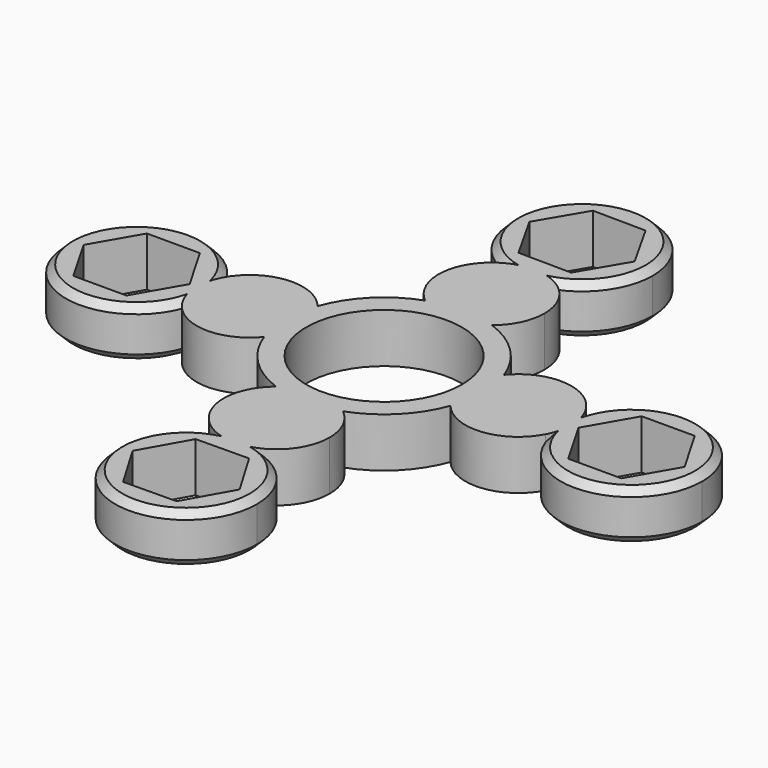
from build123d import *

# Parameters (mm, degrees)
F0_R         = 11
F1_DEPTH     = 7
F2_T4_ANGLE  = 348.6337760753
F2_S5_R      = 7.5
F2_T6_DEPTH  = 16
F2_T10_ANGLE = 348.6337760753
F2_S11_R     = 7.5
F2_T12_DEPTH = 16
F2_T16_ANGLE = 348.6337760753
F2_S17_R     = 7.5
F2_T18_DEPTH = 16
F2_T22_ANGLE = 348.6337760753
F2_S23_R     = 7.5
F2_T24_DEPTH = 16
F3_T4_ANGLE  = 348.6337760753
F3_S5_R      = 7.5
F3_T6_DEPTH  = 16
F3_T10_ANGLE = 348.6337760753
F3_S11_R     = 7.5
F3_T12_DEPTH = 16
F3_T16_ANGLE = 348.6337760753
F3_S17_R     = 7.5
F3_T18_DEPTH = 16
F3_T22_ANGLE = 348.6337760753
F3_S23_R     = 7.5
F3_T24_DEPTH = 16


# Not quite as in the source:
# - a fillet or chamfer that OpenCascade refuses, or shapes differently, is made with other operations: its cross-section is extruded or revolved along the edge and cut away or added


with BuildPart() as f1:
    # F0 (on Top) → F1 (new body)
    with BuildSketch(Plane.XY):
        with BuildLine():
            ThreePointArc((13.1776315789, -4.727581408), (13.7928757354, -2.3992871748), (14, 0))
            ThreePointArc((14, 0), (13.7928757354, 2.3992871748), (13.1776315789, 4.727581408))
            ThreePointArc((13.1776315789, 4.727581408), (11.5, 0), (13.1776315789, -4.727581408))
        make_face()
        with BuildLine():
            ThreePointArc((13.1776315789, 4.727581408), (13.7928757354, 2.3992871748), (14, 0))
            ThreePointArc((14, 0), (13.7928757354, -2.3992871748), (13.1776315789, -4.727581408))
            ThreePointArc((13.1776315789, -4.727581408), (19.7351433448, -7.4638839931), (25.6328125, -3.5008282363))
            ThreePointArc((25.6328125, -3.5008282363), (25, 0), (25.6328125, 3.5008282363))
            ThreePointArc((25.6328125, 3.5008282363), (19.7351433448, 7.4638839931), (13.1776315789, 4.727581408))
        make_face()
        with BuildLine():
            ThreePointArc((13.1776315789, -4.727581408), (11.5, 0), (13.1776315789, 4.727581408))
            ThreePointArc((13.1776315789, 4.727581408), (9.8994949366, 9.8994949366), (4.727581408, 13.1776315789))
            ThreePointArc((4.727581408, 13.1776315789), (0, 11.5), (-4.727581408, 13.1776315789))
            ThreePointArc((-4.727581408, 13.1776315789), (-9.8994949366, 9.8994949366), (-13.1776315789, 4.727581408))
            ThreePointArc((-13.1776315789, 4.727581408), (-11.9318402976, 2.5082102027), (-11.5, 0))
            ThreePointArc((-11.5, 0), (-11.9318402976, -2.5082102027), (-13.1776315789, -4.727581408))
            ThreePointArc((-13.1776315789, -4.727581408), (-9.8994949366, -9.8994949366), (-4.727581408, -13.1776315789))
            ThreePointArc((-4.727581408, -13.1776315789), (0, -11.5), (4.727581408, -13.1776315789))
            ThreePointArc((4.727581408, -13.1776315789), (9.8994949366, -9.8994949366), (13.1776315789, -4.727581408))
        make_face()
        Circle(F0_R, mode=Mode.SUBTRACT)
        with BuildLine():
            ThreePointArc((-4.727581408, 13.1776315789), (0, 11.5), (4.727581408, 13.1776315789))
            ThreePointArc((4.727581408, 13.1776315789), (0, 14), (-4.727581408, 13.1776315789))
        make_face()
        with BuildLine():
            ThreePointArc((-4.727581408, 13.1776315789), (0, 14), (4.727581408, 13.1776315789))
            ThreePointArc((4.727581408, 13.1776315789), (6.7715160991, 15.7756287869), (7.5, 19))
            ThreePointArc((7.5, 19), (6.4228580777, 22.8725823573), (3.5008282363, 25.6328125))
            ThreePointArc((3.5008282363, 25.6328125), (0, 25), (-3.5008282363, 25.6328125))
            ThreePointArc((-3.5008282363, 25.6328125), (-7.4638839931, 19.7351433448), (-4.727581408, 13.1776315789))
        make_face()
        with BuildLine():
            ThreePointArc((45, 0), (36.7787811838, 9.8405252655), (25.6328125, 3.5008282363))
            ThreePointArc((25.6328125, 3.5008282363), (26.2799757469, 1.8033172558), (26.5, 0))
            ThreePointArc((26.5, 0), (26.2799757469, -1.8033172558), (25.6328125, -3.5008282363))
            ThreePointArc((25.6328125, -3.5008282363), (36.7787811838, -9.8405252655), (45, 0))
        make_face()
        Polygon((31.2446139721, 6.4984928341), (38.7501668667, 6.5015061182), (42.5055528946, 0.0030132841), (38.7553860279, -6.4984928341), (31.2498331333, -6.5015061182), (27.4944471054, -0.0030132841), align=None, mode=Mode.SUBTRACT)
        with BuildLine():
            ThreePointArc((26.5, 0), (26.2799757469, 1.8033172558), (25.6328125, 3.5008282363))
            ThreePointArc((25.6328125, 3.5008282363), (25, 0), (25.6328125, -3.5008282363))
            ThreePointArc((25.6328125, -3.5008282363), (26.2799757469, -1.8033172558), (26.5, 0))
        make_face()
        with BuildLine():
            ThreePointArc((7.5, -19), (6.7715160991, -15.7756287869), (4.727581408, -13.1776315789))
            ThreePointArc((4.727581408, -13.1776315789), (0, -14), (-4.727581408, -13.1776315789))
            ThreePointArc((-4.727581408, -13.1776315789), (-7.4638839931, -19.7351433448), (-3.5008282363, -25.6328125))
            ThreePointArc((-3.5008282363, -25.6328125), (0, -25), (3.5008282363, -25.6328125))
            ThreePointArc((3.5008282363, -25.6328125), (6.4228580777, -22.8725823573), (7.5, -19))
        make_face()
        with BuildLine():
            ThreePointArc((-4.727581408, -13.1776315789), (0, -14), (4.727581408, -13.1776315789))
            ThreePointArc((4.727581408, -13.1776315789), (0, -11.5), (-4.727581408, -13.1776315789))
        make_face()
        with BuildLine():
            ThreePointArc((-11.5, 0), (-11.9318402976, 2.5082102027), (-13.1776315789, 4.727581408))
            ThreePointArc((-13.1776315789, 4.727581408), (-14, 0), (-13.1776315789, -4.727581408))
            ThreePointArc((-13.1776315789, -4.727581408), (-11.9318402976, -2.5082102027), (-11.5, 0))
        make_face()
        with BuildLine():
            ThreePointArc((-13.1776315789, -4.727581408), (-14, 0), (-13.1776315789, 4.727581408))
            ThreePointArc((-13.1776315789, 4.727581408), (-19.7351433448, 7.4638839931), (-25.6328125, 3.5008282363))
            ThreePointArc((-25.6328125, 3.5008282363), (-25.1594747345, 1.7787811838), (-25, 0))
            ThreePointArc((-25, 0), (-25.1594747345, -1.7787811838), (-25.6328125, -3.5008282363))
            ThreePointArc((-25.6328125, -3.5008282363), (-19.7351433448, -7.4638839931), (-13.1776315789, -4.727581408))
        make_face()
        with BuildLine():
            ThreePointArc((10, 35), (-5.7005139083, 43.216090383), (-3.5008282363, 25.6328125))
            ThreePointArc((-3.5008282363, 25.6328125), (0, 26.5), (3.5008282363, 25.6328125))
            ThreePointArc((3.5008282363, 25.6328125), (8.216090383, 29.2994860917), (10, 35))
        make_face()
        Polygon((-3.684923821, 41.5387055115), (3.8202231703, 41.4605903958), (7.5051469914, 34.9218848843), (3.684923821, 28.4612944885), (-3.8202231703, 28.5394096042), (-7.5051469914, 35.0781151157), align=None, mode=Mode.SUBTRACT)
        with BuildLine():
            ThreePointArc((3.5008282363, 25.6328125), (0, 26.5), (-3.5008282363, 25.6328125))
            ThreePointArc((-3.5008282363, 25.6328125), (0, 25), (3.5008282363, 25.6328125))
        make_face()
        with BuildLine():
            ThreePointArc((3.5008282363, -25.6328125), (0, -25), (-3.5008282363, -25.6328125))
            ThreePointArc((-3.5008282363, -25.6328125), (0, -26.5), (3.5008282363, -25.6328125))
        make_face()
        with BuildLine():
            ThreePointArc((3.5008282363, -25.6328125), (0, -26.5), (-3.5008282363, -25.6328125))
            ThreePointArc((-3.5008282363, -25.6328125), (-5.7005139083, -43.216090383), (10, -35))
            ThreePointArc((10, -35), (8.216090383, -29.2994860917), (3.5008282363, -25.6328125))
        make_face()
        Polygon((3.8202231703, -41.4605903958), (-3.684923821, -41.5387055115), (-7.5051469914, -35.0781151157), (-3.8202231703, -28.5394096042), (3.684923821, -28.4612944885), (7.5051469914, -34.9218848843), align=None, mode=Mode.SUBTRACT)
        with BuildLine():
            ThreePointArc((-25, 0), (-25.1594747345, 1.7787811838), (-25.6328125, 3.5008282363))
            ThreePointArc((-25.6328125, 3.5008282363), (-26.5, 0), (-25.6328125, -3.5008282363))
            ThreePointArc((-25.6328125, -3.5008282363), (-25.1594747345, -1.7787811838), (-25, 0))
        make_face()
        with BuildLine():
            ThreePointArc((-25.6328125, -3.5008282363), (-26.5, 0), (-25.6328125, 3.5008282363))
            ThreePointArc((-25.6328125, 3.5008282363), (-45, 0), (-25.6328125, -3.5008282363))
        make_face()
        Polygon((-38.7501668667, 6.5015061182), (-31.2446139721, 6.4984928341), (-27.4944471054, -0.0030132841), (-31.2498331333, -6.5015061182), (-38.7553860279, -6.4984928341), (-42.5055528946, 0.0030132841), align=None, mode=Mode.SUBTRACT)
    extrude(amount=F1_DEPTH)

    # F2: chamfer of 1 on 4 edges, made by hand


with BuildPart() as f2_tool2:
    # F2_s3 → F2_t4 (revolve)
    with BuildSketch(Plane(origin=(-0.3432183296, 3.4488900698, 0), x_dir=(0, 0, 1), z_dir=(0.099026451, -0.9950848014, 0))):
        Polygon((6, 24.8279680496), (7, 25.8279680496), (7, 24.8279680496), align=None)
    revolve(axis=Axis((-35, 0, 7), (0, 0, 1)), revolution_arc=F2_T4_ANGLE)

    # F2_s5 → F2_t6 (cut, symmetric)
    with BuildSketch(Plane.XY.offset(6.5)):
        with Locations((-19, 0)):
            Circle(F2_S5_R)
    extrude(amount=F2_T6_DEPTH, both=True, mode=Mode.SUBTRACT)


with BuildPart() as f1_1:
    add(f1.part)

    # F2_t1: cut F2_tool2
    add(f2_tool2.part, mode=Mode.SUBTRACT)


with BuildPart() as f2_tool8:
    # F2_s9 → F2_t10 (revolve)
    with BuildSketch(Plane(origin=(3.4488900698, 0.3432183296, 0), x_dir=(0, 0, 1), z_dir=(-0.9950848014, -0.099026451, 0))):
        Polygon((6, 24.8279680496), (7, 25.8279680496), (7, 24.8279680496), align=None)
    revolve(axis=Axis((0, 35, 7), (0, 0, 1)), revolution_arc=F2_T10_ANGLE)

    # F2_s11 → F2_t12 (cut, symmetric)
    with BuildSketch(Plane.XY.offset(6.5)):
        with Locations((0, 19)):
            Circle(F2_S11_R)
    extrude(amount=F2_T12_DEPTH, both=True, mode=Mode.SUBTRACT)


with BuildPart() as f1_2:
    add(f1_1.part)

    # F2_t7: cut F2_tool8
    add(f2_tool8.part, mode=Mode.SUBTRACT)


with BuildPart() as f2_tool14:
    # F2_s15 → F2_t16 (revolve)
    with BuildSketch(Plane(origin=(-3.4488900698, -0.3432183296, 0), x_dir=(0, 0, 1), z_dir=(0.9950848014, 0.099026451, 0))):
        Polygon((6, 24.8279680496), (7, 25.8279680496), (7, 24.8279680496), align=None)
    revolve(axis=Axis((0, -35, 7), (0, 0, 1)), revolution_arc=F2_T16_ANGLE)

    # F2_s17 → F2_t18 (cut, symmetric)
    with BuildSketch(Plane.XY.offset(6.5)):
        with Locations((0, -19)):
            Circle(F2_S17_R)
    extrude(amount=F2_T18_DEPTH, both=True, mode=Mode.SUBTRACT)


with BuildPart() as f1_3:
    add(f1_2.part)

    # F2_t13: cut F2_tool14
    add(f2_tool14.part, mode=Mode.SUBTRACT)


with BuildPart() as f2_tool20:
    # F2_s21 → F2_t22 (revolve)
    with BuildSketch(Plane(origin=(0.3432183296, -3.4488900698, 0), x_dir=(0, 0, 1), z_dir=(-0.099026451, 0.9950848014, 0))):
        Polygon((6, 24.8279680496), (7, 25.8279680496), (7, 24.8279680496), align=None)
    revolve(axis=Axis((35, 0, 7), (0, 0, 1)), revolution_arc=F2_T22_ANGLE)

    # F2_s23 → F2_t24 (cut, symmetric)
    with BuildSketch(Plane.XY.offset(6.5)):
        with Locations((19, 0)):
            Circle(F2_S23_R)
    extrude(amount=F2_T24_DEPTH, both=True, mode=Mode.SUBTRACT)


with BuildPart() as f1_4:
    add(f1_3.part)

    # F2_t19: cut F2_tool20
    add(f2_tool20.part, mode=Mode.SUBTRACT)

    # F3: chamfer of 1 on 4 edges, made by hand


with BuildPart() as f3_tool2:
    # F3_s3 → F3_t4 (revolve)
    with BuildSketch(Plane(origin=(-0.3432183296, 3.4488900698, 0), x_dir=(0, 0, 1), z_dir=(0.099026451, -0.9950848014, 0))):
        Polygon((0, 25.8279680496), (1, 24.8279680496), (0, 24.8279680496), align=None)
    revolve(axis=Axis((-35, 0, 0), (0, 0, 1)), revolution_arc=F3_T4_ANGLE)

    # F3_s5 → F3_t6 (cut, symmetric)
    with BuildSketch(Plane.XY.offset(0.5)):
        with Locations((-19, 0)):
            Circle(F3_S5_R)
    extrude(amount=F3_T6_DEPTH, both=True, mode=Mode.SUBTRACT)


with BuildPart() as f1_5:
    add(f1_4.part)

    # F3_t1: cut F3_tool2
    add(f3_tool2.part, mode=Mode.SUBTRACT)


with BuildPart() as f3_tool8:
    # F3_s9 → F3_t10 (revolve)
    with BuildSketch(Plane(origin=(-3.4488900698, -0.3432183296, 0), x_dir=(0, 0, 1), z_dir=(0.9950848014, 0.099026451, 0))):
        Polygon((0, 25.8279680496), (1, 24.8279680496), (0, 24.8279680496), align=None)
    revolve(axis=Axis((0, -35, 0), (0, 0, 1)), revolution_arc=F3_T10_ANGLE)

    # F3_s11 → F3_t12 (cut, symmetric)
    with BuildSketch(Plane.XY.offset(0.5)):
        with Locations((0, -19)):
            Circle(F3_S11_R)
    extrude(amount=F3_T12_DEPTH, both=True, mode=Mode.SUBTRACT)


with BuildPart() as f1_6:
    add(f1_5.part)

    # F3_t7: cut F3_tool8
    add(f3_tool8.part, mode=Mode.SUBTRACT)


with BuildPart() as f3_tool14:
    # F3_s15 → F3_t16 (revolve)
    with BuildSketch(Plane(origin=(0.3432183296, -3.4488900698, 0), x_dir=(0, 0, 1), z_dir=(-0.099026451, 0.9950848014, 0))):
        Polygon((1, 24.8279680496), (0, 25.8279680496), (0, 24.8279680496), align=None)
    revolve(axis=Axis((35, 0, 0), (0, 0, 1)), revolution_arc=F3_T16_ANGLE)

    # F3_s17 → F3_t18 (cut, symmetric)
    with BuildSketch(Plane.XY.offset(0.5)):
        with Locations((19, 0)):
            Circle(F3_S17_R)
    extrude(amount=F3_T18_DEPTH, both=True, mode=Mode.SUBTRACT)


with BuildPart() as f1_7:
    add(f1_6.part)

    # F3_t13: cut F3_tool14
    add(f3_tool14.part, mode=Mode.SUBTRACT)


with BuildPart() as f3_tool20:
    # F3_s21 → F3_t22 (revolve)
    with BuildSketch(Plane(origin=(3.4488900698, 0.3432183296, 0), x_dir=(0, 0, 1), z_dir=(-0.9950848014, -0.099026451, 0))):
        Polygon((0, 25.8279680496), (1, 24.8279680496), (0, 24.8279680496), align=None)
    revolve(axis=Axis((0, 35, 0), (0, 0, 1)), revolution_arc=F3_T22_ANGLE)

    # F3_s23 → F3_t24 (cut, symmetric)
    with BuildSketch(Plane.XY.offset(0.5)):
        with Locations((0, 19)):
            Circle(F3_S23_R)
    extrude(amount=F3_T24_DEPTH, both=True, mode=Mode.SUBTRACT)


with BuildPart() as f1_8:
    add(f1_7.part)

    # F3_t19: cut F3_tool20
    add(f3_tool20.part, mode=Mode.SUBTRACT)


solid = f1_8.part
